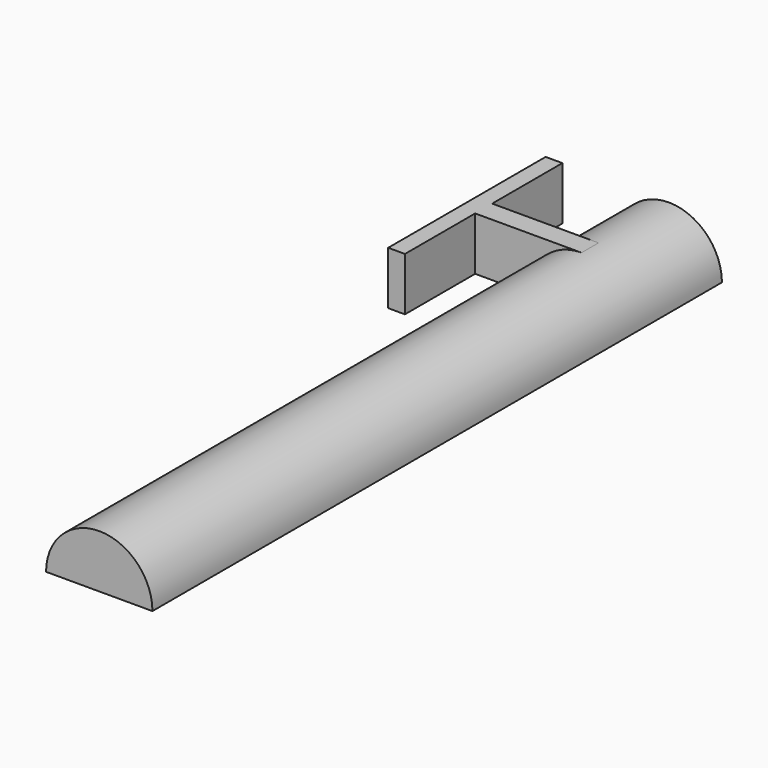
from build123d import *

# Parameters (mm, degrees)
F1_DEPTH = 170
F2_W     = 25.4
F2_H     = 5.08
F3_DEPTH = 12.7
F4_W     = 20.96
F4_H     = 12.7
F4_W_2   = 2.54
F5_DEPTH = 4


with BuildPart() as f1:
    # F0 (on Front) → F1 (new body)
    with BuildSketch(Plane.XZ):
        with BuildLine():
            Line((-12.7, 0), (12.7, 0))
            ThreePointArc((12.7, 0), (0, 12.7), (-12.7, 0))
        make_face()
    extrude(amount=F1_DEPTH)

    # F2 (on face) → F3 (join)
    with BuildSketch(Plane(origin=(0, 0, 0), x_dir=(1, 0, 0), z_dir=(0, 0, -1))):
        with Locations((-12.7, 23.5)):
            Rectangle(F2_W, F2_H)
    extrude(amount=-F3_DEPTH)

    # F4 (on face) → F5 (join)
    with BuildSketch(Plane(origin=(-25.4, 0, 0), x_dir=(0, -1, 0), z_dir=(-1, 0, 0))):
        with Locations((36.52, 6.35)):
            Rectangle(F4_W, F4_H)
        with Locations((10.48, 6.35)):
            Rectangle(F4_W, F4_H)
        with Locations((22.23, 6.35)):
            Rectangle(F4_W_2, F4_H)
        with Locations((24.77, 6.35)):
            Rectangle(F4_W_2, F4_H)
    extrude(amount=F5_DEPTH)


solid = f1.part
